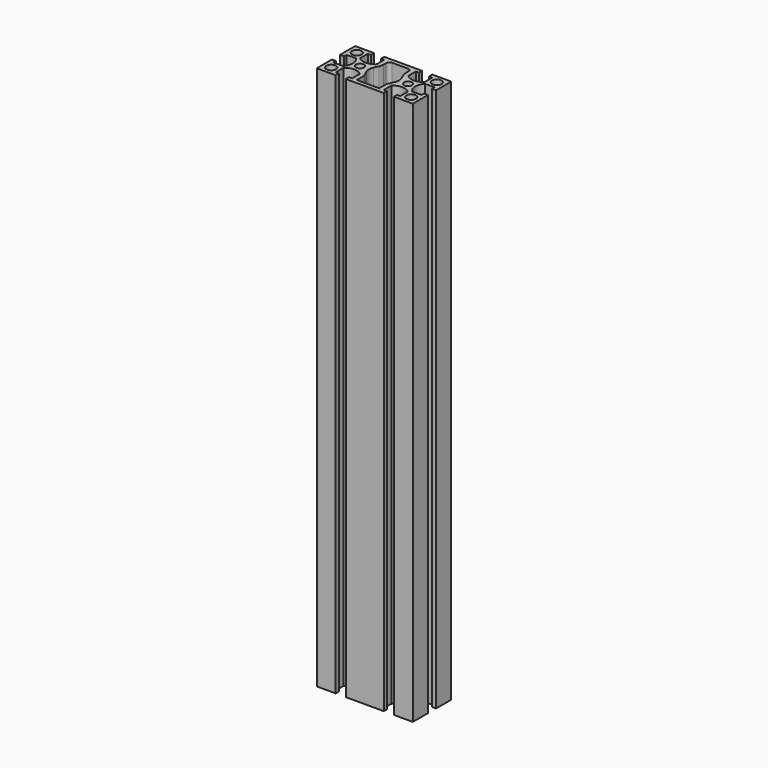
from build123d import *

# Parameters (mm, degrees)
F0_R     = 3
F0_R_2   = 2.5
F1_DEPTH = 340
F2_R     = 2
F3_R     = 7


# Not quite as in the source:
# - a feature names something its author has since deleted; it is built from what else it names


with BuildPart() as f1:
    # F0 (on Top) → F1 (new body)
    with BuildSketch(Plane.XY):
        with BuildLine():
            Line((18.15, -15), (30, -15))
            Line((30, -15), (30, -3.15))
            Line((30, -3.15), (27.5, -3.15))
            Line((27.5, -3.15), (27.5, -5.15))
            Line((27.5, -5.15), (21.5477069044, -5.15))
            ThreePointArc((21.5477069044, -5.15), (19.5, 0), (21.5477069044, 5.15))
            Line((21.5477069044, 5.15), (27.5, 5.15))
            Line((27.5, 5.15), (27.5, 3.15))
            Line((27.5, 3.15), (30, 3.15))
            Line((30, 3.15), (30, 15))
            Line((30, 15), (18.15, 15))
            Line((18.15, 15), (18.15, 12.5))
            Line((18.15, 12.5), (20.15, 12.5))
            Line((20.15, 12.5), (20.15, 6.5477069044))
            ThreePointArc((20.15, 6.5477069044), (15, 4.5), (9.85, 6.5477069044))
            Line((9.85, 6.5477069044), (9.85, 12.5))
            Line((9.85, 12.5), (11.85, 12.5))
            Line((11.85, 12.5), (11.85, 15))
            Line((11.85, 15), (-11.85, 15))
            Line((-11.85, 15), (-11.85, 12.5))
            Line((-11.85, 12.5), (-9.85, 12.5))
            Line((-9.85, 12.5), (-9.85, 6.5477069044))
            ThreePointArc((-9.85, 6.5477069044), (-15, 4.5), (-20.15, 6.5477069044))
            Line((-20.15, 6.5477069044), (-20.15, 12.5))
            Line((-20.15, 12.5), (-18.15, 12.5))
            Line((-18.15, 12.5), (-18.15, 15))
            Line((-18.15, 15), (-30, 15))
            Line((-30, 15), (-30, 3.15))
            Line((-30, 3.15), (-27.5, 3.15))
            Line((-27.5, 3.15), (-27.5, 5.15))
            Line((-27.5, 5.15), (-21.5477069044, 5.15))
            ThreePointArc((-21.5477069044, 5.15), (-19.5, 0), (-21.5477069044, -5.15))
            Line((-21.5477069044, -5.15), (-27.5, -5.15))
            Line((-27.5, -5.15), (-27.5, -3.15))
            Line((-27.5, -3.15), (-30, -3.15))
            Line((-30, -3.15), (-30, -15))
            Line((-30, -15), (-18.15, -15))
            Line((-18.15, -15), (-18.15, -12.5))
            Line((-18.15, -12.5), (-20.15, -12.5))
            Line((-20.15, -12.5), (-20.15, -6.5477069044))
            ThreePointArc((-20.15, -6.5477069044), (-15, -4.5), (-9.85, -6.5477069044))
            Line((-9.85, -6.5477069044), (-9.85, -12.5))
            Line((-9.85, -12.5), (-11.85, -12.5))
            Line((-11.85, -12.5), (-11.85, -15))
            Line((-11.85, -15), (11.85, -15))
            Line((11.85, -15), (11.85, -12.5))
            Line((11.85, -12.5), (9.85, -12.5))
            Line((9.85, -12.5), (9.85, -6.5477069044))
            ThreePointArc((9.85, -6.5477069044), (15, -4.5), (20.15, -6.5477069044))
            Line((20.15, -6.5477069044), (20.15, -12.5))
            Line((20.15, -12.5), (18.15, -12.5))
            Line((18.15, -12.5), (18.15, -15))
        make_face()
        with Locations((-25, -10)):
            Circle(F0_R, mode=Mode.SUBTRACT)
        with Locations((25, -10)):
            Circle(F0_R, mode=Mode.SUBTRACT)
        with Locations((-15, 0)):
            Circle(F0_R_2, mode=Mode.SUBTRACT)
        with Locations((-25, 10)):
            Circle(F0_R, mode=Mode.SUBTRACT)
        Polygon((-7, 7), (-7, 12.5), (0, 12.5), (7, 12.5), (7, 7), (10, 0), (7, -7), (7, -12.5), (0, -12.5), (-7, -12.5), (-7, -7), (-10, 0), align=None, mode=Mode.SUBTRACT)
        with Locations((15, 0)):
            Circle(F0_R_2, mode=Mode.SUBTRACT)
        with Locations((25, 10)):
            Circle(F0_R, mode=Mode.SUBTRACT)
    extrude(amount=F1_DEPTH)

    # F2
    f2_edges = [f1.edges().sort_by_distance(p)[0] for p in [
        (-7, 12.5, 170),
        (7, 12.5, 170),
    ]]
    fillet(f2_edges, radius=F2_R)

    # F3
    f3_edges = [f1.edges().sort_by_distance(p)[0] for p in [
        (-7, 7, 170),
        (-10, 0, 170),
        (7, 7, 170),
        (10, 0, 170),
    ]]
    fillet(f3_edges, radius=F3_R)


solid = f1.part
